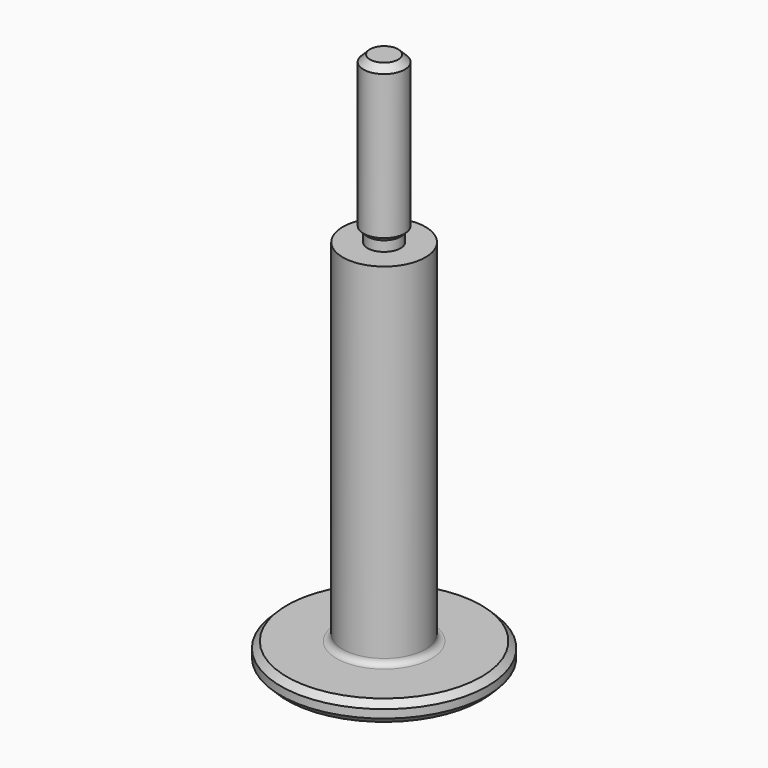
from build123d import *

# Parameters (mm, degrees)
F2_R        = 1.5
F3_SIZE     = 1.5
F4_S7_R     = 4
F4_T8_DEPTH = 9


# Not quite as in the source:
# - a fillet or chamfer that OpenCascade refuses, or shapes differently, is made with other operations: its cross-section is extruded or revolved along the edge and cut away or added


with BuildPart() as f1:
    # F0 (on Front) → F1 (revolve)
    with BuildSketch(Plane.XZ):
        Polygon((0, 130), (0, 0), (25, 0), (25, 5), (10, 5), (10, 90), (4, 90), (4, 91.8505489826), (5, 91.8505489826), (5, 130), align=None)
    revolve(axis=Axis((0, 0, 65), (0, 0, 1)))

    # F2
    f2_edges = [f1.edges().sort_by_distance(p)[0] for p in [
        (-10, 0, 5),
    ]]
    fillet(f2_edges, radius=F2_R)

    # F3
    f3_edges = [f1.edges().sort_by_distance(p)[0] for p in [
        (-25, 0, 5),
        (-25, 0, 0),
    ]]
    chamfer(f3_edges, length=F3_SIZE)

    # F4: chamfer of 1.6 on 2 edges, made by hand

    # F4_s1 → F4_t2 (revolve, cut)
    with BuildSketch(Plane.XZ):
        Polygon((5, 128.4), (3.4, 130), (5, 130), align=None)
    revolve(axis=Axis((0, 0, 130), (0, 0, 1)), mode=Mode.SUBTRACT)


with BuildPart() as f4_tool4:
    # F4_s5 → F4_t6 (revolve)
    with BuildSketch(Plane.XZ):
        Polygon((3.4, 91.8505489826), (5, 93.4505489826), (5, 91.8505489826), align=None)
    revolve(axis=Axis((0, 0, 91.8505489826), (0, 0, 1)))

    # F4_s7 → F4_t8 (cut, symmetric)
    with BuildSketch(Plane.XY.offset(92.7)):
        Circle(F4_S7_R)
    extrude(amount=F4_T8_DEPTH, both=True, mode=Mode.SUBTRACT)


with BuildPart() as f1_1:
    add(f1.part)

    # F4_t3: cut F4_tool4
    add(f4_tool4.part, mode=Mode.SUBTRACT)


solid = f1_1.part
